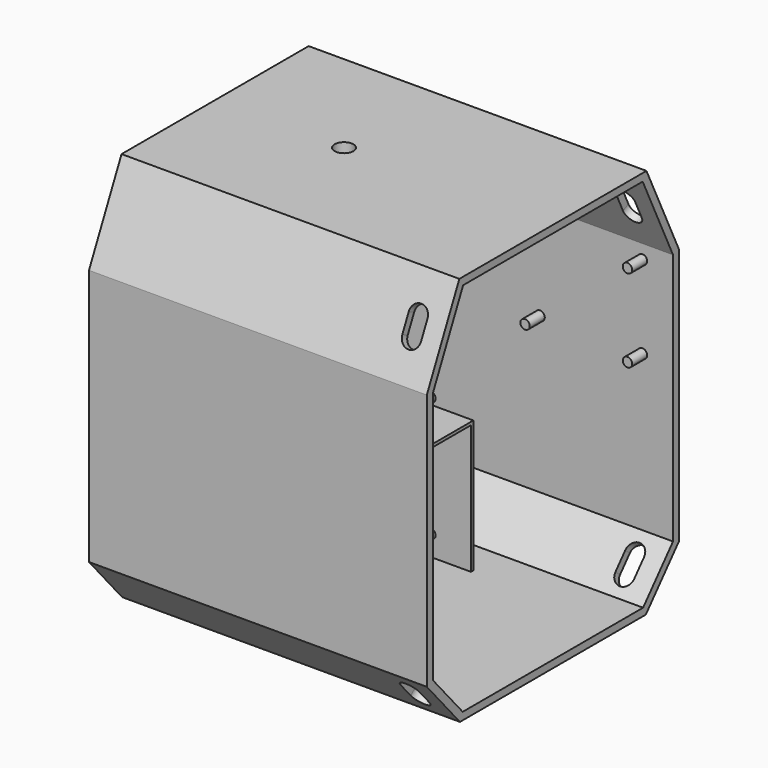
from build123d import *

# Parameters (mm, degrees)
F1_DEPTH  = 2.54
F2_DEPTH  = 114.3
F3_R      = 1.5875
F4_DEPTH  = 6.35
F6_DEPTH  = 63.45
F7_R      = 1.5875
F8_DEPTH  = 6.35
F9_R      = 1.5875
F10_DEPTH = 6.35
F12_DEPTH = 12.7
F13_DEPTH = 25.4
F15_DEPTH = 25.4
F17_DEPTH = 25.4
F18_W     = 53.5
F18_H     = 37.5681460026
F19_DEPTH = 2.54
F21_R     = 5.08
F21_R_2   = 3.175
F22_DEPTH = 12.7
F23_R     = 3.175
F24_DEPTH = 25.4


# Not quite as in the source:
# - a pattern or mirror of a feature is missing from the dataset's text; its kind, count and spacing are read off the source's solid


with BuildPart() as f1:
    # F0 (on Right) → F1 (new body)
    with BuildSketch(Plane.YZ):
        Polygon((53.34, 24.4303685296), (39.5708099851, 53.4414463806), (-39.5708099851, 53.4414463806), (-53.34, 24.4303685296), (-53.34, -62.4677875109), (-39.3094271421, -78.6385536194), (39.3094271421, -78.6385536194), (53.34, -62.4677875109), align=None)
        Polygon((-50.8, -61.5194703762), (-50.8, 23.8581906473), (-37.9647744794, 50.9014463806), (37.9647744794, 50.9014463806), (50.8, 23.8581906473), (50.8, -61.5194703762), (38.1504515326, -76.0985536194), (-38.1504515326, -76.0985536194), align=None, mode=Mode.SUBTRACT)
        Polygon((-37.9647744794, 50.9014463806), (-50.8, 23.8581906473), (-50.8, -61.5194703762), (-38.1504515326, -76.0985536194), (38.1504515326, -76.0985536194), (50.8, -61.5194703762), (50.8, 23.8581906473), (37.9647744794, 50.9014463806), align=None)
    extrude(amount=F1_DEPTH)

    # F0 (on Right) → F2 (join)
    with BuildSketch(Plane.YZ):
        Polygon((53.34, 24.4303685296), (39.5708099851, 53.4414463806), (-39.5708099851, 53.4414463806), (-53.34, 24.4303685296), (-53.34, -62.4677875109), (-39.3094271421, -78.6385536194), (39.3094271421, -78.6385536194), (53.34, -62.4677875109), align=None)
        Polygon((-50.8, -61.5194703762), (-50.8, 23.8581906473), (-37.9647744794, 50.9014463806), (37.9647744794, 50.9014463806), (50.8, 23.8581906473), (50.8, -61.5194703762), (38.1504515326, -76.0985536194), (-38.1504515326, -76.0985536194), align=None, mode=Mode.SUBTRACT)
    extrude(amount=F2_DEPTH)

    # F3 (on face) → F4 (join)
    with BuildSketch(Plane.YZ.offset(2.54)):
        with Locations((-22.4663, 44.4899889485)):
            Circle(F3_R)
        with Locations((22.4663, 44.4899889485)):
            Circle(F3_R)
        with Locations((22.4663, 11.4445889485)):
            Circle(F3_R)
        with Locations((-22.4663, 11.4445889485)):
            Circle(F3_R)
    extrude(amount=F4_DEPTH)

    # F5 (on face) → F6 (join)
    with BuildSketch(Plane.YZ.offset(2.54)):
        Polygon((-26.75, -31.3985536194), (-26.75, -76.0985536194), (-25.75, -76.0985536194), (-25.75, -32.3985536194), (25.75, -32.3985536194), (25.75, -76.0985536194), (26.75, -76.0985536194), (26.75, -31.3985536194), align=None)
    extrude(amount=F6_DEPTH)

    # F7 (on face) → F8 (join)
    with BuildSketch(Plane(origin=(0, -50.8, 0), x_dir=(-1, 0, 0), z_dir=(0, 1, 0))):
        with Locations((-108.5821617321, 18.4301891438)):
            Circle(F7_R)
        with Locations((-108.5821617321, -22.3368108562)):
            Circle(F7_R)
        with Locations((-42.6437617321, -22.3368108562)):
            Circle(F7_R)
        with Locations((-42.6437617321, 18.4301891438)):
            Circle(F7_R)
    extrude(amount=F8_DEPTH)

    # F9 (on face) → F10 (join)
    with BuildSketch(Plane.XZ.offset(-50.8)):
        with Locations((103.9661599512, 19.124702289)):
            Circle(F9_R)
        with Locations((69.3205599512, 19.124702289)):
            Circle(F9_R)
        with Locations((69.3205599512, -8.891497711)):
            Circle(F9_R)
        with Locations((103.9661599512, -8.891497711)):
            Circle(F9_R)
    extrude(amount=F10_DEPTH)

    # F11 (on face) → F12 (join)
    with BuildSketch(Plane.YZ.offset(2.54)):
        Polygon((-49.8278358551, -62.639926338), (-45.9908042053, -59.3107240133), (-37.6677983936, -68.9033031377), (-41.5048300434, -72.2325054624), (-40.6725294623, -73.1917633748), (-35.8762399, -69.030260469), (-45.8638468741, -57.5191655197), (-50.6601364363, -61.6806684255), align=None)
        Polygon((-50.8, 1.4893601356), (-50.8, 0.2193601356), (-45.72, 0.2193601356), (-45.72, -37.8806398644), (-50.8, -37.8806398644), (-50.8, -39.1506398644), (-44.45, -39.1506398644), (-44.45, 1.4893601356), align=None)
        Polygon((-38.3923937628, 50.0004713555), (-38.9369386243, 48.853139279), (-34.3476103183, 46.6749598328), (-45.2385075491, 23.7283183028), (-49.8278358551, 25.9064977489), (-50.3723807167, 24.7591656724), (-44.6357203341, 22.0364413647), (-32.6557333803, 47.2777470478), align=None)
        Polygon((44.45, 1.4893601356), (44.45, -39.1506398644), (50.8, -39.1506398644), (50.8, -37.8806398644), (45.72, -37.8806398644), (45.72, 0.2193601356), (50.8, 0.2193601356), (50.8, 1.4893601356), align=None)
        Polygon((40.6725294623, -73.1917633748), (41.5048300434, -72.2325054624), (37.6677983936, -68.9033031377), (45.9908042053, -59.3107240133), (49.8278358551, -62.639926338), (50.6601364363, -61.6806684255), (45.8638468741, -57.5191655197), (35.8762399, -69.030260469), align=None)
        Polygon((49.8278358551, 25.9064977489), (45.2385075491, 23.7283183028), (34.3476103183, 46.6749598328), (38.9369386243, 48.853139279), (38.3923937628, 50.0004713555), (32.6557333803, 47.2777470478), (44.6357203341, 22.0364413647), (50.3723807167, 24.7591656724), align=None)
    extrude(amount=F12_DEPTH)

    # F13 (cut): faces of the model
    f13_faces = [f1.faces().sort_by_distance(p)[0] for p in [
        (2.54, -42.0877230867, 36.2907287909),
        (2.54, -48.26, -18.8306398644),
        (2.54, 48.26, -18.8306398644),
        (2.54, 42.0877230867, 36.2907287909),
        (2.54, 43.7478171244, -65.7716147378),
        (2.54, -43.7478171244, -65.7716147378),
    ]]
    extrude(f13_faces, amount=-F13_DEPTH, mode=Mode.SUBTRACT)

    # F14 (on face) → F15 (cut)
    with BuildSketch(Plane(origin=(0, 52.9968859392, 25.1532947669), x_dir=(-1, 0, 0), z_dir=(0, 0.9034110839, 0.4287754815))):
        with BuildLine():
            Line((-101.6, 12.0811917099), (-101.6, 18.4311917099))
            ThreePointArc((-101.6, 18.4311917099), (-104.775, 21.6061917099), (-107.95, 18.4311917099))
            Line((-107.95, 18.4311917099), (-107.95, 12.0811917099))
            ThreePointArc((-107.95, 12.0811917099), (-104.775, 8.9061917099), (-101.6, 12.0811917099))
        make_face()
    f15 = extrude(amount=-F15_DEPTH, mode=Mode.SUBTRACT)

    # F15_copies: F15 across plane
    add(f15.mirror(Plane(origin=(0, 0, 0), x_dir=(0, 0, -1), z_dir=(0, -1, 0))), mode=Mode.SUBTRACT)

    # F16 (on face) → F17 (cut)
    with BuildSketch(Plane(origin=(0, 61.3527734682, -53.2327629009), x_dir=(-1, 0, 0), z_dir=(0, 0.7553211909, -0.6553547883))):
        with BuildLine():
            Line((-101.6, -26.1061819567), (-101.6, -19.7561819567))
            ThreePointArc((-101.6, -19.7561819567), (-104.775, -16.5811819567), (-107.95, -19.7561819567))
            Line((-107.95, -19.7561819567), (-107.95, -26.1061819567))
            ThreePointArc((-107.95, -26.1061819567), (-104.775, -29.2811819567), (-101.6, -26.1061819567))
        make_face()
    f17 = extrude(amount=-F17_DEPTH, mode=Mode.SUBTRACT)

    # F17_copies: F17 across plane
    add(f17.mirror(Plane(origin=(0, 0, 0), x_dir=(0, 0, -1), z_dir=(0, -1, 0))), mode=Mode.SUBTRACT)

    # F18 (on face) → F19 (cut)
    with BuildSketch(Plane(origin=(0, 0, 0), x_dir=(0, -1, 0), z_dir=(-1, 0, 0))):
        with Locations((0, -12.6144806181)):
            Rectangle(F18_W, F18_H)
    extrude(amount=-F19_DEPTH, mode=Mode.SUBTRACT)

    # F21 (on face) → F22 (join)
    with BuildSketch(Plane.XY.offset(53.4414463806)):
        with Locations((43.6254143715, 0)):
            Circle(F21_R)
        with Locations((43.6254143715, 0)):
            Circle(F21_R_2, mode=Mode.SUBTRACT)
    extrude(amount=-F22_DEPTH)

    # F23 (on face) → F24 (cut)
    with BuildSketch(Plane.XY.offset(53.4414463806)):
        with Locations((43.6254143715, 0)):
            Circle(F23_R)
    extrude(amount=-F24_DEPTH, mode=Mode.SUBTRACT)


solid = f1.part
